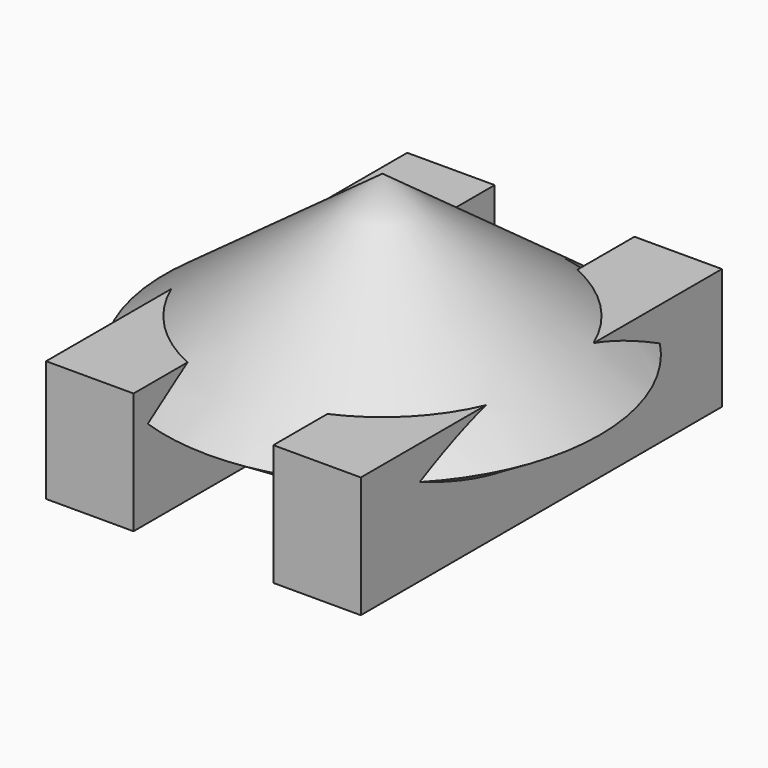
from build123d import *

# Parameters (mm, degrees)
F2_W     = 29.6725835651
F2_H     = 153.1317234039
F3_DEPTH = 41.148


# Not quite as in the source:
# - the program builds the solid bodies; features that only make, move or delete a surface that nothing else refers to are left out


with BuildPart() as f1:
    # F0 (on Front) → F1 (revolve)
    with BuildSketch(Plane.XZ):
        Polygon((0, 42.5218716264), (0, -38.5478623211), (44.3764105439, -29.5401159674), (73.7840533257, -11.5246195346), align=None)
    revolve(axis=Axis((0, 0, 1.9870046526), (0, 0, -1)))

    # F2 (on Top) → F3 (join)
    with BuildSketch(Plane.XY):
        with Locations((-38.5478632525, 0.6623342633)):
            Rectangle(F2_W, F2_H)
        with Locations((38.5478632525, 0.6623342633)):
            Rectangle(F2_W, F2_H)
    extrude(amount=-F3_DEPTH)


solid = f1.part
